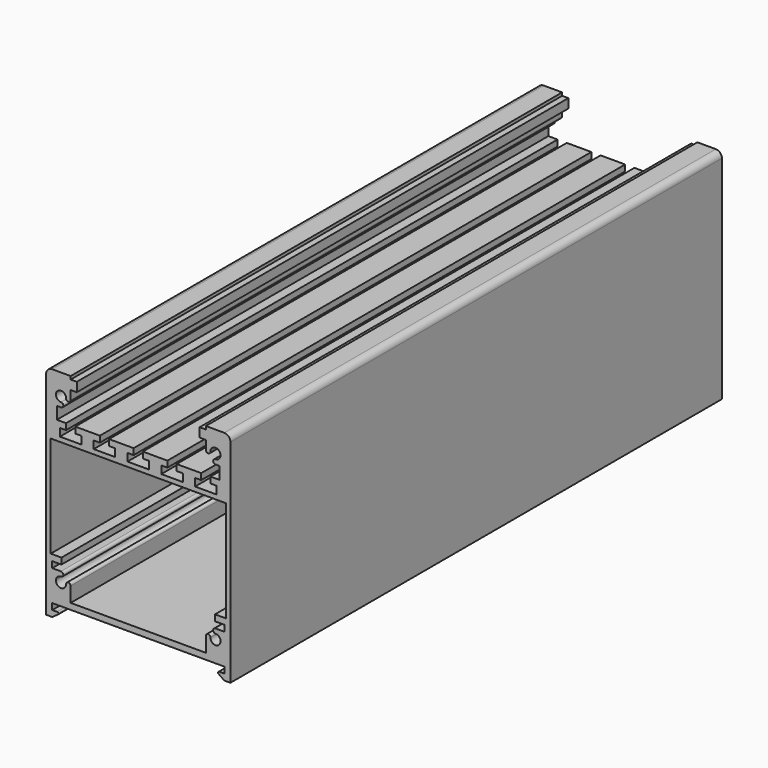
from build123d import *

# Parameters (mm, degrees)
F1_DEPTH = 200


# Not quite as in the source:
# - ends of sketch curves that miss each other by under 0.0002 mm in the source are joined


with BuildPart() as f1:
    # F0 (on Front) → F1 (new body)
    with BuildSketch(Plane.XZ):
        with BuildLine():
            Line((26.171612, -51.228388), (28, -52.5))
            Line((28, -52.5), (30, -52.5))
            Line((30, -52.5), (30, 16.5))
            ThreePointArc((30, 16.5), (29.4142135624, 17.9142135624), (28, 18.5))
            Line((28, 18.5), (22, 18.5))
            Line((22, 18.5), (22, 17.5))
            Line((22, 17.5), (20, 17.5))
            Line((20, 17.5), (20, 14.5))
            Line((20, 14.5), (22, 14.5))
            Line((22, 14.5), (22, 11.643728))
            ThreePointArc((22, 11.643728), (22.746864, 10.896864), (23.493728, 11.643728))
            ThreePointArc((23.493728, 11.643728), (26.310454189, 12.810454189), (25.143728, 9.993728))
            ThreePointArc((25.143728, 9.993728), (24.396864, 9.246864), (25.143728, 8.5))
            Line((25.143728, 8.5), (26.5, 8.5))
            Line((26.5, 8.5), (26.5, 4.5))
            Line((26.5, 4.5), (23.5, 4.5))
            Line((23.5, 4.5), (23.5, 2.5))
            Line((23.5, 2.5), (25.5, 2.5))
            Line((25.5, 2.5), (25.5, 0))
            Line((25.5, 0), (18.5, 0))
            Line((18.5, 0), (18.5, 2.5))
            Line((18.5, 2.5), (20.5, 2.5))
            Line((20.5, 2.5), (20.5, 4.5))
            Line((20.5, 4.5), (12.5, 4.5))
            Line((12.5, 4.5), (12.5, 2.5))
            Line((12.5, 2.5), (14.5, 2.5))
            Line((14.5, 2.5), (14.5, 0))
            Line((14.5, 0), (7.5, 0))
            Line((7.5, 0), (7.5, 2.5))
            Line((7.5, 2.5), (9.5, 2.5))
            Line((9.5, 2.5), (9.5, 4.5))
            Line((9.5, 4.5), (1.5, 4.5))
            Line((1.5, 4.5), (1.5, 2.5))
            Line((1.5, 2.5), (3.5, 2.5))
            Line((3.5, 2.5), (3.5, 0))
            Line((3.5, 0), (-3.5, 0))
            Line((-3.5, 0), (-3.5, 2.5))
            Line((-3.5, 2.5), (-1.5, 2.5))
            Line((-1.5, 2.5), (-1.5, 4.5))
            Line((-1.5, 4.5), (-9.5, 4.5))
            Line((-9.5, 4.5), (-9.5, 2.5))
            Line((-9.5, 2.5), (-7.5, 2.5))
            Line((-7.5, 2.5), (-7.5, 0))
            Line((-7.5, 0), (-14.5, 0))
            Line((-14.5, 0), (-14.5, 2.5))
            Line((-14.5, 2.5), (-12.5, 2.5))
            Line((-12.5, 2.5), (-12.5, 4.5))
            Line((-12.5, 4.5), (-20.5, 4.5))
            Line((-20.5, 4.5), (-20.5, 2.5))
            Line((-20.5, 2.5), (-18.5, 2.5))
            Line((-18.5, 2.5), (-18.5, 0))
            Line((-18.5, 0), (-25.5, 0))
            Line((-25.5, 0), (-25.5, 2.5))
            Line((-25.5, 2.5), (-23.5, 2.5))
            Line((-23.5, 2.5), (-23.5, 4.5))
            Line((-23.5, 4.5), (-26.5, 4.5))
            Line((-26.5, 4.5), (-26.5, 8.5))
            Line((-26.5, 8.5), (-25.143728, 8.5))
            ThreePointArc((-25.143728, 8.5), (-24.396864, 9.246864), (-25.143728, 9.993728))
            ThreePointArc((-25.143728, 9.993728), (-26.310454189, 12.810454189), (-23.493728, 11.643728))
            ThreePointArc((-23.493728, 11.643728), (-22.746864, 10.896864), (-22, 11.643728))
            Line((-22, 11.643728), (-22, 14.5))
            Line((-22, 14.5), (-20, 14.5))
            Line((-20, 14.5), (-20, 17.5))
            Line((-20, 17.5), (-22, 17.5))
            Line((-22, 17.5), (-22, 18.5))
            Line((-22, 18.5), (-28, 18.5))
            ThreePointArc((-28, 18.5), (-29.4142135624, 17.9142135624), (-30, 16.5))
            Line((-30, 16.5), (-30, -52.5))
            Line((-30, -52.5), (-28, -52.5))
            Line((-28, -52.5), (-26.171612, -51.228388))
            ThreePointArc((-26.171612, -51.228388), (-26.0454895845, -51.0852629626), (-26, -50.9))
            ThreePointArc((-26, -50.9), (-26.1171572875, -50.6171572875), (-26.4, -50.5))
            Line((-26.4, -50.5), (-28, -50.5))
            Line((-28, -50.5), (-28, -48.5))
            Line((-28, -48.5), (28, -48.5))
            Line((28, -48.5), (28, -50.5))
            Line((28, -50.5), (26.4, -50.5))
            ThreePointArc((26.4, -50.5), (26.1171572875, -50.6171572875), (26, -50.9))
            ThreePointArc((26, -50.9), (26.0454895845, -51.0852629626), (26.171612, -51.228388))
        make_face()
        with BuildLine():
            Line((-22, -46.5), (-22, -41.643728))
            ThreePointArc((-22, -41.643728), (-22.746864, -40.896864), (-23.493728, -41.643728))
            ThreePointArc((-23.493728, -41.643728), (-26.310454189, -42.810454189), (-25.143728, -39.993728))
            ThreePointArc((-25.143728, -39.993728), (-24.396864, -39.246864), (-25.143728, -38.5))
            Line((-25.143728, -38.5), (-28, -38.5))
            Line((-28, -38.5), (-28, -36.5))
            Line((-28, -36.5), (-25, -36.5))
            Line((-25, -36.5), (-25, -34.5))
            Line((-25, -34.5), (-28.5, -34.5))
            Line((-28.5, -34.5), (-28.5, -1.5))
            Line((-28.5, -1.5), (28.5, -1.5))
            Line((28.5, -1.5), (28.5, -34.5))
            Line((28.5, -34.5), (25, -34.5))
            Line((25, -34.5), (25, -36.5))
            Line((25, -36.5), (28, -36.5))
            Line((28, -36.5), (28, -38.5))
            Line((28, -38.5), (25.143728, -38.5))
            ThreePointArc((25.143728, -38.5), (24.396864, -39.246864), (25.143728, -39.993728))
            ThreePointArc((25.143728, -39.993728), (26.310454189, -42.810454189), (23.493728, -41.643728))
            ThreePointArc((23.493728, -41.643728), (22.746864, -40.896864), (22, -41.643728))
            Line((22, -41.643728), (22, -46.5))
            Line((22, -46.5), (-22, -46.5))
        make_face(mode=Mode.SUBTRACT)
    extrude(amount=F1_DEPTH)


solid = f1.part
